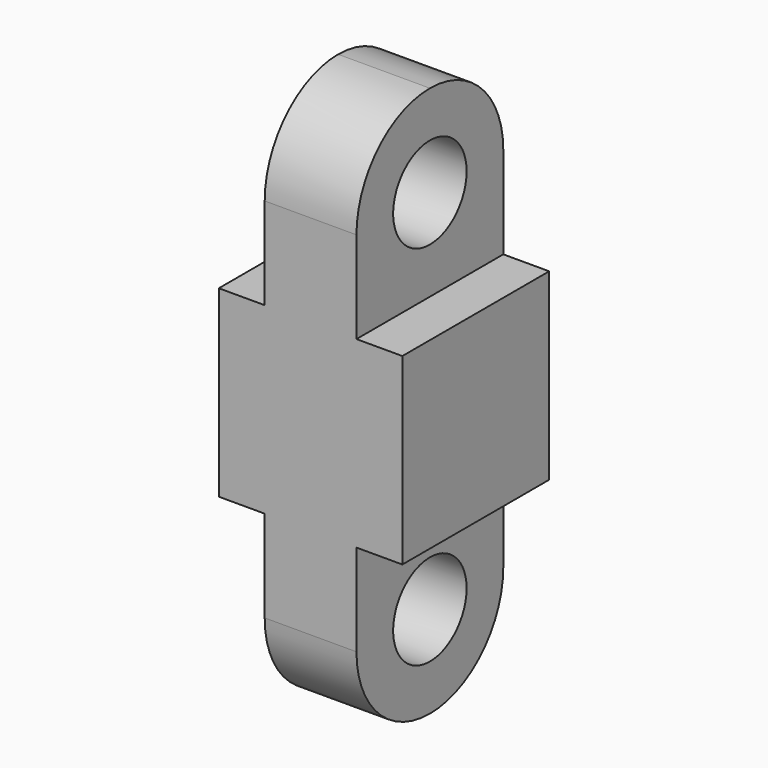
from build123d import *

# Parameters (mm, degrees)
F0_W     = 20
F0_H     = 20
F1_DEPTH = 40
F2_R     = 19.99999
F3_R     = 10
F5_DEPTH = 20
F4_R     = 10
F6_DEPTH = 20


# Not quite as in the source:
# - a fillet or chamfer is up to 0.001 mm smaller than in the source, because OpenCascade refuses the exact size


with BuildPart() as f1:
    # F0 (on Front) → F1 (new body)
    with BuildSketch(Plane.XZ):
        Polygon((10, -20), (20, -20), (20, 20), (10, 20), (-10, 20), (-20, 20), (-20, -20), (-10, -20), (-10, -40), (10, -40), align=None)
        with Locations((0, 30)):
            Rectangle(F0_W, F0_H)
        with Locations((0, 50)):
            Rectangle(F0_W, F0_H)
        with Locations((0, -50)):
            Rectangle(F0_W, F0_H)
    extrude(amount=F1_DEPTH)

    # F2 (radius 20 in the source; OpenCascade refuses exactly that, so slightly less here)
    f2_edges = [f1.edges().sort_by_distance(p)[0] for p in [
        (0, -40, 60),
        (0, 0, 60),
        (0, -40, -60),
        (0, 0, -60),
    ]]
    fillet(f2_edges, radius=F2_R)

    # F3 (on face) → F5 (cut, through all)
    with BuildSketch(Plane.YZ.offset(10)):
        with Locations((-20, 40)):
            Circle(F3_R)
    extrude(amount=-F5_DEPTH, mode=Mode.SUBTRACT)

    # F4 (on face) → F6 (cut, through all)
    with BuildSketch(Plane.YZ.offset(10)):
        with Locations((-20, -40)):
            Circle(F4_R)
    extrude(amount=-F6_DEPTH, mode=Mode.SUBTRACT)


solid = f1.part
